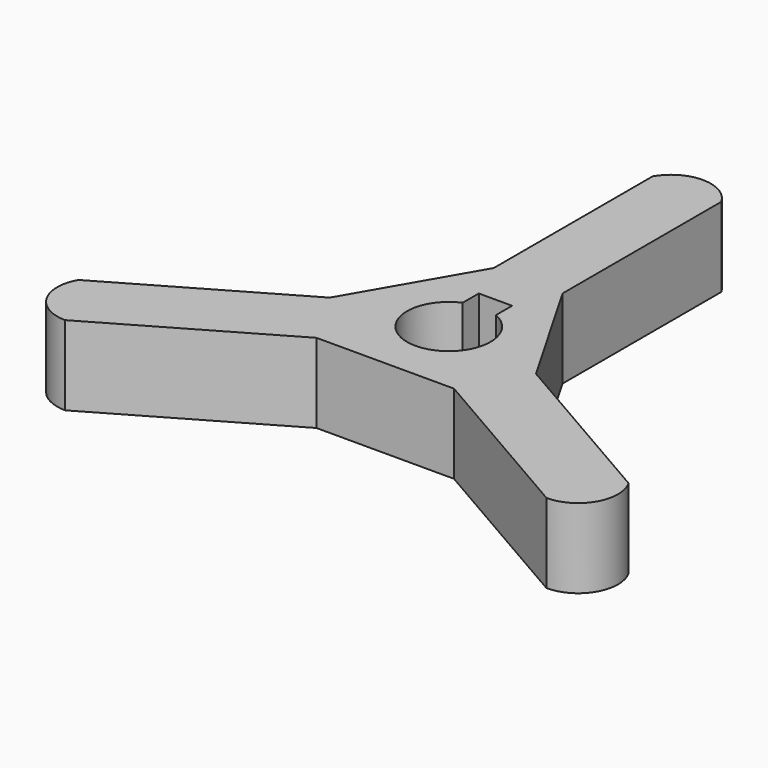
from build123d import *

# Parameters (mm, degrees)
F2_DEPTH = 9.525


# Not quite as in the source:
# - a variable given as a bare number and used for a length is read in inches; the dataset says mm whatever the document's units were


with BuildPart() as f2:
    # F1 (on Top) → F2 (new body)
    with BuildSketch(Plane.XY):
        with BuildLine():
            Line((4.1244459855, 11.90625), (4.1244459855, 35.71875))
            ThreePointArc((4.1244459855, 35.71875), (0, 38.1), (-4.1244459855, 35.71875))
            Line((-4.1244459855, 35.71875), (-4.1244459855, 11.90625))
            Line((-4.1244459855, 11.90625), (0, 19.05))
            Line((0, 19.05), (4.1244459855, 11.90625))
        make_face()
        with BuildLine():
            Line((4.1244459855, 7.14375), (4.1244459855, 11.90625))
            Line((4.1244459855, 11.90625), (0, 19.05))
            Line((0, 19.05), (0, 7))
            Line((0, 7), (2, 7))
            Line((2, 7), (2, 4.582575695))
            ThreePointArc((2, 4.582575695), (4.1833001327, 2.7386127875), (5, 0))
            ThreePointArc((5, 0), (4.8296291314, -1.2940952255), (4.3301270189, -2.5))
            Line((4.3301270189, -2.5), (16.4977839421, -9.525))
            Line((16.4977839421, -9.525), (12.3733379566, -2.38125))
            Line((12.3733379566, -2.38125), (8.248891971, 0))
            Line((8.248891971, 0), (4.1244459855, 7.14375))
        make_face()
        with BuildLine():
            Line((0, 19.05), (-4.1244459855, 11.90625))
            Line((-4.1244459855, 11.90625), (-4.1244459855, 7.14375))
            Line((-4.1244459855, 7.14375), (-8.248891971, 0))
            Line((-8.248891971, 0), (-12.3733379566, -2.38125))
            Line((-12.3733379566, -2.38125), (-16.4977839421, -9.525))
            Line((-16.4977839421, -9.525), (-4.3301270189, -2.5))
            ThreePointArc((-4.3301270189, -2.5), (-4.7495627838, 1.562579074), (-2, 4.582575695))
            Line((-2, 4.582575695), (-2, 7))
            Line((-2, 7), (0, 7))
            Line((0, 7), (0, 19.05))
        make_face()
        with BuildLine():
            Line((4.1244459855, -7.14375), (8.248891971, -9.525))
            Line((8.248891971, -9.525), (16.4977839421, -9.525))
            Line((16.4977839421, -9.525), (4.3301270189, -2.5))
            ThreePointArc((4.3301270189, -2.5), (0, -5), (-4.3301270189, -2.5))
            Line((-4.3301270189, -2.5), (-16.4977839421, -9.525))
            Line((-16.4977839421, -9.525), (-8.248891971, -9.525))
            Line((-8.248891971, -9.525), (-4.1244459855, -7.14375))
            Line((-4.1244459855, -7.14375), (4.1244459855, -7.14375))
        make_face()
        with BuildLine():
            ThreePointArc((28.8711218987, -21.43125), (32.9955678842, -19.05), (32.9955678842, -14.2875))
            Line((32.9955678842, -14.2875), (12.3733379566, -2.38125))
            Line((12.3733379566, -2.38125), (16.4977839421, -9.525))
            Line((16.4977839421, -9.525), (8.248891971, -9.525))
            Line((8.248891971, -9.525), (28.8711218987, -21.43125))
        make_face()
        with BuildLine():
            Line((-12.3733379566, -2.38125), (-32.9955678842, -14.2875))
            ThreePointArc((-32.9955678842, -14.2875), (-32.9955678842, -19.05), (-28.8711218987, -21.43125))
            Line((-28.8711218987, -21.43125), (-8.248891971, -9.525))
            Line((-8.248891971, -9.525), (-16.4977839421, -9.525))
            Line((-16.4977839421, -9.525), (-12.3733379566, -2.38125))
        make_face()
        Polygon((-8.248891971, -9.525), (8.248891971, -9.525), (4.1244459855, -7.14375), (-4.1244459855, -7.14375), align=None)
        Polygon((12.3733379566, -2.38125), (4.1244459855, 11.90625), (4.1244459855, 7.14375), (8.248891971, 0), align=None)
        Polygon((-4.1244459855, 7.14375), (-4.1244459855, 11.90625), (-12.3733379566, -2.38125), (-8.248891971, 0), align=None)
    extrude(amount=F2_DEPTH)


solid = f2.part
